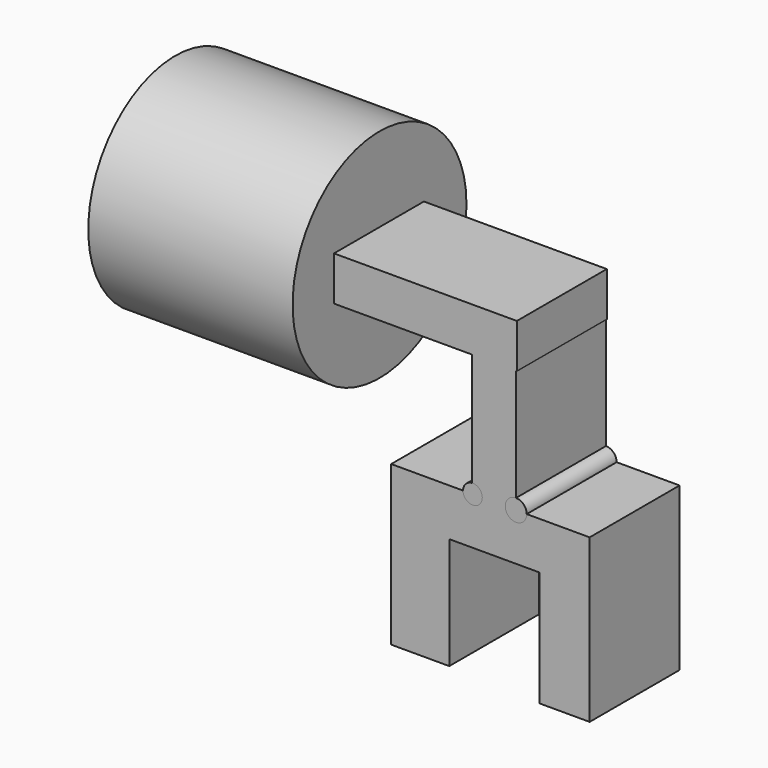
from build123d import *

# Parameters (mm, degrees)
F0_W     = 9.9890101701
F0_H     = 27.7146026492
F0_W_2   = 13.1228137761
F0_H_2   = 25.2663148567
F0_W_3   = 11.3600492477
F0_H_3   = 26.0497657582
F2_DEPTH = 25.4
F1_R     = 2.4246663919
F1_R_2   = 2.1744313886
F4_R     = 24.5610859867
F5_DEPTH = 46.17845


# Not quite as in the source:
# - a feature of the source that left no trace in its solid (it failed there, or was rolled back) is left out


with BuildPart() as f2:
    # F0 (on Front) → F2 (new body)
    with BuildSketch(Plane.XZ):
        Polygon((41.3270741701, 37.7036109567), (-46.2236478925, 37.7036109567), (-46.2236478925, 27.7146026492), (31.1422031373, 27.7146026492), (41.1312133074, 27.7146026492), (41.3270741701, 27.7146026492), align=None)
        with Locations((36.1367082223, 13.8573013246)):
            Rectangle(F0_W, F0_H)
        Polygon((41.1312133074, 0), (31.1422031373, 0), (12.9269529134, 0), (12.9269529134, -10.6745297089), (26.0497666895, -10.6745297089), (46.4195124805, -10.6745297089), (57.7795617282, -10.6745297089), (57.7795617282, 0), align=None)
        with Locations((19.4883598015, -23.3076871373)):
            Rectangle(F0_W_2, F0_H_2)
        with Locations((52.0995371044, -23.699412588)):
            Rectangle(F0_W_3, F0_H_3)
    extrude(amount=F2_DEPTH)

    # F4 (on Right) → F5 (join)
    with BuildSketch(Plane.YZ):
        with Locations((-12.5352256, 32.2194471955)):
            Circle(F4_R)
    extrude(amount=-F5_DEPTH)


with BuildPart() as f2b:
    # F1 (on Front) → F2, piece 2 (new body)
    with BuildSketch(Plane.XZ):
        with Locations((41.1312133074, 0)):
            Circle(F1_R)
    extrude(amount=F2_DEPTH)


with BuildPart() as f2c:
    # F1 (on Front) → F2, piece 3 (new body)
    with BuildSketch(Plane.XZ):
        with Locations((31.3380658627, 0)):
            Circle(F1_R_2)
    extrude(amount=F2_DEPTH)


solid = Compound([f2.part, f2b.part, f2c.part])
